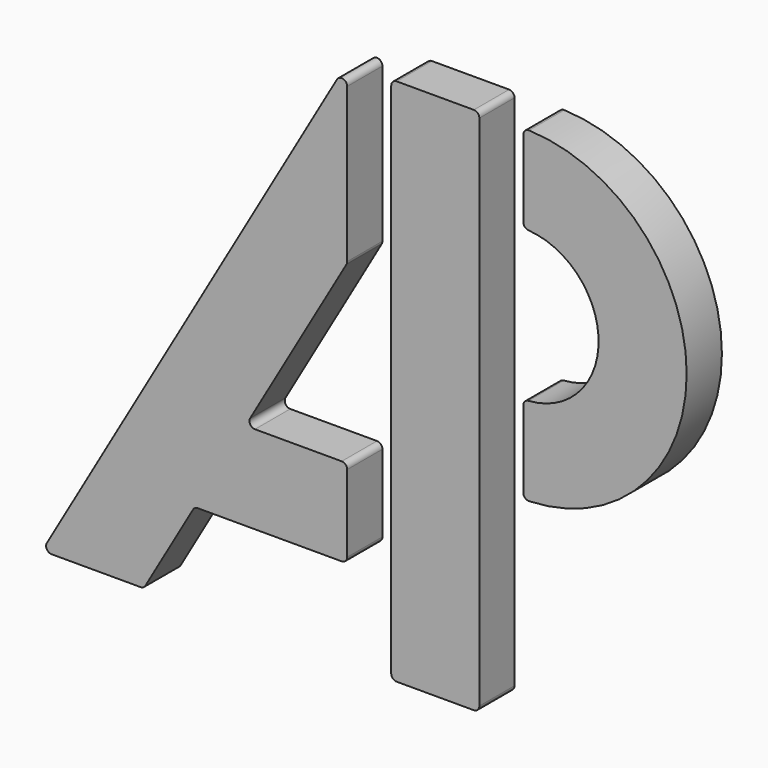
from build123d import *

# Parameters (mm, degrees)
F2_DEPTH = 6.35
F3_R     = 0.79375
F3_2_R   = 0.79375
F3_3_R   = 0.79375


# Not quite as in the source:
# - a variable given as a bare number and used for a length is read in inches; the dataset says mm whatever the document's units were


with BuildPart() as f2:
    # F1 (on Front) → F2 (new body)
    with BuildSketch(Plane.XZ):
        Polygon((-12.7, 12.7), (-12.7, 38.1), (-56.6940905122, -38.1), (-42.0293936748, -38.1), (-34.6970452561, -25.4), (-27.3646968374, -12.7), align=None)
        Polygon((-12.7, -25.4), (-12.7, -12.7), (-27.3646968374, -12.7), (-34.6970452561, -25.4), align=None)
    extrude(amount=F2_DEPTH)

    # F3
    f3_edges = [f2.edges().sort_by_distance(p)[0] for p in [
        (-12.7, -3.175, 38.1),
        (-12.7, -3.175, 12.7),
        (-12.7, -3.175, -25.4),
        (-34.697045, -3.175, -25.4),
        (-42.029394, -3.175, -38.1),
        (-56.694091, -3.175, -38.1),
        (-27.364697, -3.175, -12.7),
        (-12.7, -3.175, -12.7),
    ]]
    fillet(f3_edges, radius=F3_R)


with BuildPart() as f2b:
    # F1 (on Front) → F2, piece 2 (new body)
    with BuildSketch(Plane.XZ):
        Polygon((6.35, 38.1), (-6.35, 38.1), (-6.35, 12.7), (-6.35, -12.7), (-6.35, -25.4), (-6.35, -38.1), (6.35, -38.1), (6.35, -8.9941899428), (6.35, 3.7058100572), (6.35, 25.4), align=None)
    extrude(amount=F2_DEPTH)

    # F3#2
    f3_2_edges = [f2b.edges().sort_by_distance(p)[0] for p in [
        (-6.35, -3.175, 38.1),
        (6.35, -3.175, 38.1),
        (-6.35, -3.175, -38.1),
        (6.35, -3.175, -38.1),
    ]]
    fillet(f3_2_edges, radius=F3_2_R)


with BuildPart() as f2c:
    # F1 (on Front) → F2, piece 3 (new body)
    with BuildSketch(Plane.XZ):
        with BuildLine():
            ThreePointArc((12.7, -8.9941899428), (36.2470949714, 14.5529050286), (12.7, 38.1))
            Line((12.7, 38.1), (12.7, 25.4))
            ThreePointArc((12.7, 25.4), (23.5470949714, 14.5529050286), (12.7, 3.7058100572))
            Line((12.7, 3.7058100573), (12.7, -8.9941899428))
        make_face()
    extrude(amount=F2_DEPTH)

    # F3#3
    f3_3_edges = [f2c.edges().sort_by_distance(p)[0] for p in [
        (12.7, -3.175, -8.99419),
        (12.7, -3.175, 3.70581),
        (12.7, -3.175, 25.4),
        (12.7, -3.175, 38.1),
    ]]
    fillet(f3_3_edges, radius=F3_3_R)


solid = Compound([f2.part, f2b.part, f2c.part])
